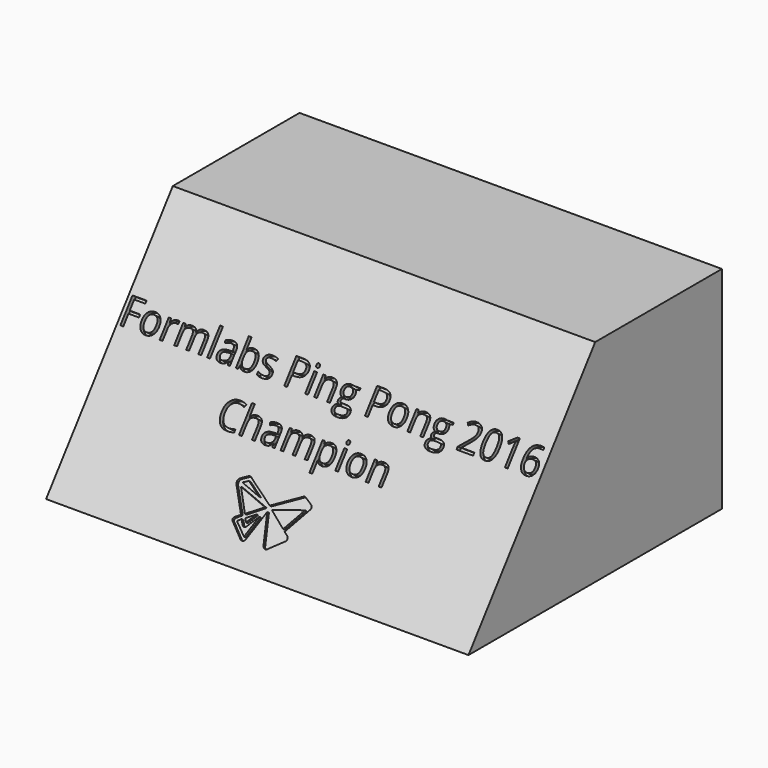
from build123d import *

# Parameters (mm, degrees)
F0_W         = 101.6
F0_H         = 76.2
F1_DEPTH     = 50.8
F3_DEPTH     = 101.601
F4_T         = -2.54
F5_TEXT_SIZE = 8.5353903059
F6_DEPTH     = 1.27
F8_DEPTH     = 0.635
F9_TEXT_SIZE = 3.5123019997
F10_DEPTH    = 1.27


# Not quite as in the source:
# - Text() gives the source's letters only with a copy of the font that has no kerning and outlines rounded to 1/6400 em; it was checked with that copy


with BuildPart() as f1:
    # F0 (on Top) → F1 (new body)
    with BuildSketch(Plane.XY):
        with Locations((16.9333308506, 38.1)):
            Rectangle(F0_W, F0_H)
    extrude(amount=F1_DEPTH)

    # F2 (on face) → F3 (cut, through all)
    with BuildSketch(Plane.YZ.offset(67.7333308506)):
        Polygon((0, 50.8), (0, 0), (38.1, 50.8), align=None)
    extrude(amount=-F3_DEPTH, mode=Mode.SUBTRACT)

    # F4
    f4_openings = [f1.faces().sort_by_distance(p)[0] for p in [
        (16.933331, 38.1, 0),
    ]]
    offset(amount=F4_T, openings=f4_openings)

    # F5 (on face) → F6 (cut)
    with BuildSketch(Plane(origin=(0, 0, 0), x_dir=(1, 0, 0), z_dir=(0, -0.8, 0.6))):
        with Locations((-33.878014423, 35.4853495955)):
            Text('Formlabs Ping Pong 2016', F5_TEXT_SIZE, font='Open Sans', text_align=(TextAlign.LEFT, TextAlign.BOTTOM))
        with Locations((-5.0457327007, 23.8772187796)):
            Text('Champion', F5_TEXT_SIZE, font='Open Sans', text_align=(TextAlign.LEFT, TextAlign.BOTTOM))
    extrude(amount=-F6_DEPTH, mode=Mode.SUBTRACT)

    # F7 (on face) → F8 (cut)
    with BuildSketch(Plane(origin=(0, 0, 0), x_dir=(1, 0, 0), z_dir=(0, -0.8, 0.6))):
        with BuildLine():
            Line((13.4837115183, 13.4272510186), (7.3560709134, 17.118493095))
            ThreePointArc((7.3560709134, 17.118493095), (6.9598628009, 17.3219317084), (6.5232547931, 17.2339454293))
            Line((6.5232547931, 17.2339454293), (5.0372248515, 16.3523033261))
            ThreePointArc((5.0372248515, 16.3523033261), (4.5941037589, 15.7553422177), (4.7088782303, 15.0208044797))
            Line((4.7088782303, 15.0208044797), (8.2500472502, 9.9444482787))
            Line((8.2500472502, 9.9444482787), (7.0838008274, 9.1308970741))
            ThreePointArc((7.0838008274, 9.1308970741), (6.8475814061, 8.6456949987), (7.1361442097, 8.1896772608))
            Line((7.1361442097, 8.1896772608), (10.2178193629, 5.5576669984))
            ThreePointArc((10.2178193629, 5.5576669984), (10.8682715637, 5.4446336831), (11.3433087245, 5.9031140991))
            Line((11.3433087245, 5.9031140991), (13.5008823127, 12.1355671436))
            Line((13.5008823127, 12.1355671436), (15.5845545232, 5.9314654209))
            ThreePointArc((15.5845545232, 5.9314654209), (15.9616371116, 5.4979932508), (16.5347233415, 5.4572308436))
            Line((16.5347233415, 5.4572308436), (19.7310019284, 8.081631735))
            ThreePointArc((19.7310019284, 8.081631735), (20.041796176, 8.6354321435), (19.7362490992, 9.1921447629))
            Line((19.7362490992, 9.1921447629), (18.8143051114, 9.7729407743))
            Line((18.8143051114, 9.7729407743), (22.2590983821, 15.2411368069))
            ThreePointArc((22.2590983821, 15.2411368069), (22.3842901343, 15.813418361), (22.0345240086, 16.2833575159))
            Line((22.0345240086, 16.2833575159), (20.3393120319, 17.2168835998))
            ThreePointArc((20.3393120319, 17.2168835998), (19.9693319663, 17.2853947372), (19.6317466821, 17.1192165172))
            Line((19.6317466821, 17.1192165172), (13.4837115183, 13.4272510186))
        make_face()
        with BuildLine():
            Line((10.2651705965, 8.0516058952), (12.2502879319, 10.7989438046))
            Line((12.2502879319, 10.7989438046), (10.7283759862, 6.2629207969))
            Line((10.7283759862, 6.2629207969), (7.9214246944, 8.5824187845))
            Line((7.9214246944, 8.5824187845), (8.7465365849, 9.2327181414))
            Line((8.7465365849, 9.2327181414), (9.4287740067, 8.2547133788))
            ThreePointArc((9.4287740067, 8.2547133788), (9.8085458541, 7.9949195314), (10.2651705965, 8.0516058952))
        make_face(mode=Mode.SUBTRACT)
        Polygon((9.4586731866, 9.6149612218), (11.4831300452, 11.0469274223), (9.9453385919, 8.9157661423), align=None, mode=Mode.SUBTRACT)
        Polygon((5.8720999334, 14.8942405851), (12.6240206882, 12.8366881981), (8.9787328616, 10.3465225548), align=None, mode=Mode.SUBTRACT)
        Polygon((5.7934536599, 15.7347135246), (7.0594344288, 16.4298992604), (10.5455731973, 14.3083883449), align=None, mode=Mode.SUBTRACT)
        Polygon((14.2554277554, 12.8213027492), (21.3006008416, 14.9052804336), (18.2668808848, 10.1485736668), align=None, mode=Mode.SUBTRACT)
    extrude(amount=-F8_DEPTH, mode=Mode.SUBTRACT)

    # F9 (on face) → F10 (cut)
    with BuildSketch(Plane.XZ.offset(-73.66)):
        with Locations((-12.3573746532, 19.5230711251)):
            Text('Designed & Printed by David Liu', F9_TEXT_SIZE, font='Open Sans', text_align=(TextAlign.LEFT, TextAlign.BOTTOM))
    extrude(amount=-F10_DEPTH, mode=Mode.SUBTRACT)


solid = f1.part
